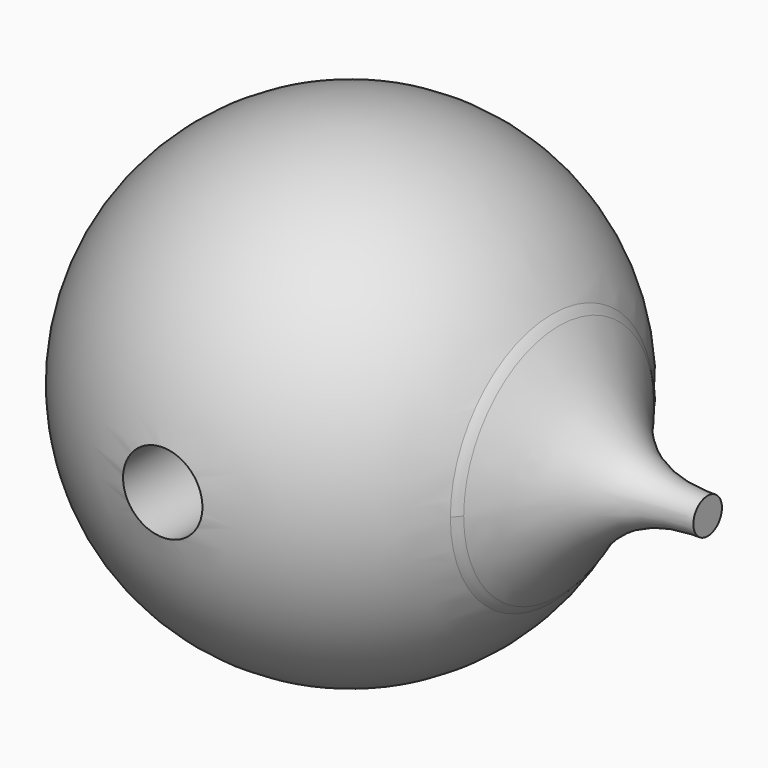
from build123d import *

# Parameters (mm, degrees)
F3_R        = 10.16
F4_DEPTH    = 15.875
F7_R        = 3.175
F8_DEPTH    = 25.4
F9_T2_ANGLE = 180.0000002199
F9_T4_ANGLE = 179.9999999345


# Not quite as in the source:
# - a fillet or chamfer that OpenCascade refuses, or shapes differently, is made with other operations: its cross-section is extruded or revolved along the edge and cut away or added


with BuildPart() as f1:
    # F0 (on Front) → F1 (revolve)
    with BuildSketch(Plane.XZ):
        with BuildLine():
            Line((0, 19.05), (0, -19.05))
            ThreePointArc((0, -19.05), (19.05, 0), (0, 19.05))
        make_face()
    revolve(axis=Axis((0, 0, 0), (0, 0, -1)))

    # F3 (on offset) → F4 (join)
    with BuildSketch(Plane.YZ.offset(12.7)):
        Circle(F3_R)
    extrude(amount=F4_DEPTH)

    # F5 (on Top) → F6 (revolve, cut)
    with BuildSketch(Plane.XY):
        with BuildLine():
            add(Edge.make_bspline(
                [(16.0334594548, -10.3644961491), (17.5619016312, -8.4434705035), (22.291404173, -0.7556150252), (28.8937536319, -1.4395783264), (30.1896631718, -1.4926075237)],
                knots=[0, 0, 0, 0, 0.5565187358, 1, 1, 1, 1], degree=3))
            Line((16.0334594548, -10.3644961491), (30.1896631718, -10.3644961491))
            Line((30.1896631718, -10.3644961491), (30.1896631718, -1.4926075237))
        make_face()
    revolve(axis=Axis((23.3597867191, 0, 0), (-1, 0, 0)), mode=Mode.SUBTRACT)

    # F7 (on Front) → F8 (cut, symmetric)
    with BuildSketch(Plane.XZ):
        Circle(F7_R)
    extrude(amount=F8_DEPTH, both=True, mode=Mode.SUBTRACT)

    # F9: fillet of radius 5.08 on 2 edges, made by hand

    # F9_s1 → F9_t2 (revolve, cut)
    with BuildSketch(Plane.XY.offset(-1.95e-08)):
        with BuildLine():
            ThreePointArc((16.1144934764, -10.1599999963), (16.407046723, -9.8527346061), (16.6729403711, -9.5221291161))
            Line((16.6729403711, -9.5221291161), (16.7547016298, -9.5824421047))
            ThreePointArc((16.7547016298, -9.5824421047), (16.5162775071, -9.9033020934), (16.2740232311, -10.2220962285))
            Line((16.2740232311, -10.2220962285), (16.1936079439, -10.2616))
            ThreePointArc((16.1936079439, -10.2616), (16.1540507101, -10.2615999963), (16.1850857971, -10.2330704024))
            Line((16.1850857971, -10.2330704024), (16.1144934764, -10.1599999963))
        make_face()
    revolve(axis=Axis((16.1936079439, -1.58e-08, -1.95e-08), (1, 0, 0)), revolution_arc=F9_T2_ANGLE, mode=Mode.SUBTRACT)

    # F9_s3 → F9_t4 (revolve, cut)
    with BuildSketch(Plane.XY.offset(-5.8e-09)):
        with BuildLine():
            ThreePointArc((16.1144934764, 10.1600000025), (16.407046723, 9.8527346123), (16.6729403711, 9.5221291223))
            Line((16.6729403711, 9.5221291223), (16.7547016298, 9.5824421109))
            ThreePointArc((16.7547016298, 9.5824421109), (16.5162775086, 9.9033020976), (16.2740232311, 10.2220962285))
            Line((16.2740232311, 10.2220962285), (16.1936079439, 10.2616))
            ThreePointArc((16.1936079439, 10.2616), (16.1540507101, 10.2616000025), (16.1850857971, 10.2330704086))
            Line((16.1850857971, 10.2330704086), (16.1144934764, 10.1600000025))
        make_face()
    revolve(axis=Axis((16.1936079439, -3.3e-09, -5.8e-09), (1, 0, 0)), revolution_arc=F9_T4_ANGLE, mode=Mode.SUBTRACT)


solid = f1.part
